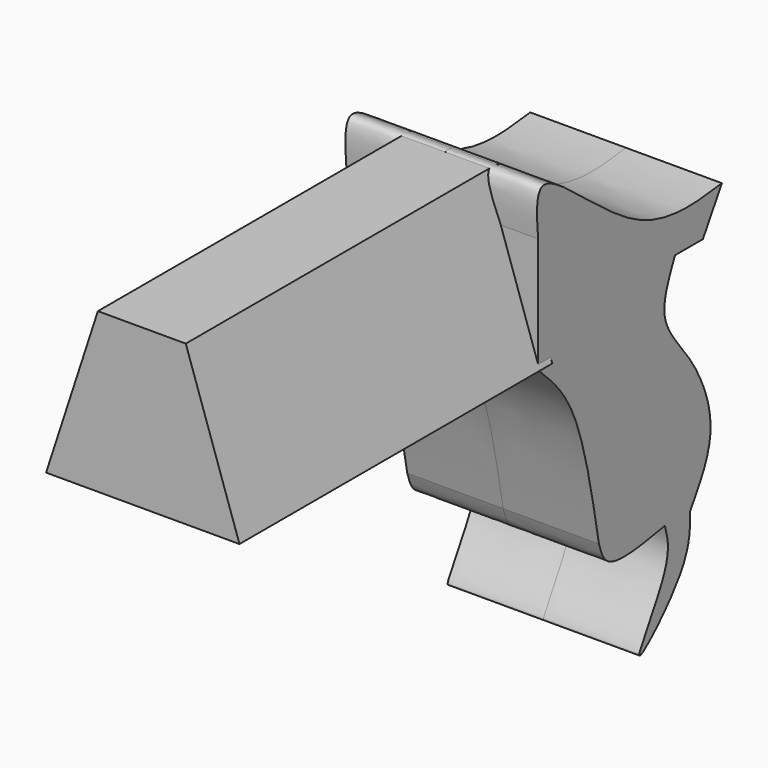
from build123d import *

# Parameters (mm, degrees)
F1_DEPTH      = 25
F1_DEPTH_BACK = 25
F3_DEPTH      = 102


with BuildPart() as f1:
    # F0 (on Right) → F1 (new body, two sides)
    with BuildSketch(Plane.YZ) as f1_sk:
        with BuildLine():
            Line((97.9158058763, 30.1268287003), (97.9158058763, 0))
            add(Edge.make_bspline(
                [(97.9158058763, 0), (101.8021663079, -3.696980686), (111.322754248, -12.7536367407), (115.3632833237, -34.8885167563), (117.7544444799, -47.9878075421)],
                knots=[0, 0, 0, 0, 0.4082059276, 1, 1, 1, 1], degree=3))
            add(Edge.make_bspline(
                [(117.7544444799, -47.9878075421), (118.3996283157, -50.1406766369), (120.140772316, -55.9505790246), (131.8659232896, -53.853910931), (139.2462998629, -52.5341667235)],
                knots=[0, 0, 0, 0, 0.3705516808, 1, 1, 1, 1], degree=3))
            add(Edge.make_bspline(
                [(139.2462998629, -52.5341667235), (140.1012876765, -55.3905852567), (142.0883412882, -62.0291088385), (123.351206173, -87.5491233148), (147.5744893106, -65.1804071235), (147.5319825692, -56.5218574441), (147.5124061108, -52.5341667235)],
                knots=[0, 0, 0, 0, 0.2075483266, 0.4823573452, 0.7615999345, 1, 1, 1, 1], degree=3))
            add(Edge.make_bspline(
                [(147.5124061108, -52.5341667235), (150.6703452653, -47.5471900273), (157.2604657803, -37.1401568881), (148.7008340103, -17.2326111997), (136.3144713941, -5.3646602758), (140.5310533356, 3.8186216049), (142.5527483225, 8.2216653973)],
                knots=[0, 0, 0, 0, 0.2547960421, 0.5317191187, 0.7754766483, 1, 1, 1, 1], degree=3))
            Line((142.5527483225, 8.2216653973), (151.6454517841, 8.2216653973))
            Line((151.6454517841, 8.2216653973), (157.8450202942, 18.5542888939))
            add(Edge.make_bspline(
                [(157.8450202942, 18.5542888939), (148.8377384911, 17.4304544494), (129.7771030879, 15.0522676591), (96.2484454593, 50.8784565164), (97.4710717705, 35.6618987099), (97.9158058763, 30.1268287003)],
                knots=[0, 0, 0, 0, 0.3630752259, 0.7683166416, 1, 1, 1, 1], degree=3))
        make_face()
    extrude(amount=F1_DEPTH)
    extrude(f1_sk.sketch, amount=-F1_DEPTH_BACK)

    # F2 (on Front) → F3 (join)
    with BuildSketch(Plane.XZ):
        Polygon((-11.4919018, 41.4746329188), (-25, 0), (0, 0), (25.4404135048, 0), (11.436519213, 41.4746329188), (0, 41.4746329188), align=None)
    extrude(amount=-F3_DEPTH)


solid = f1.part
